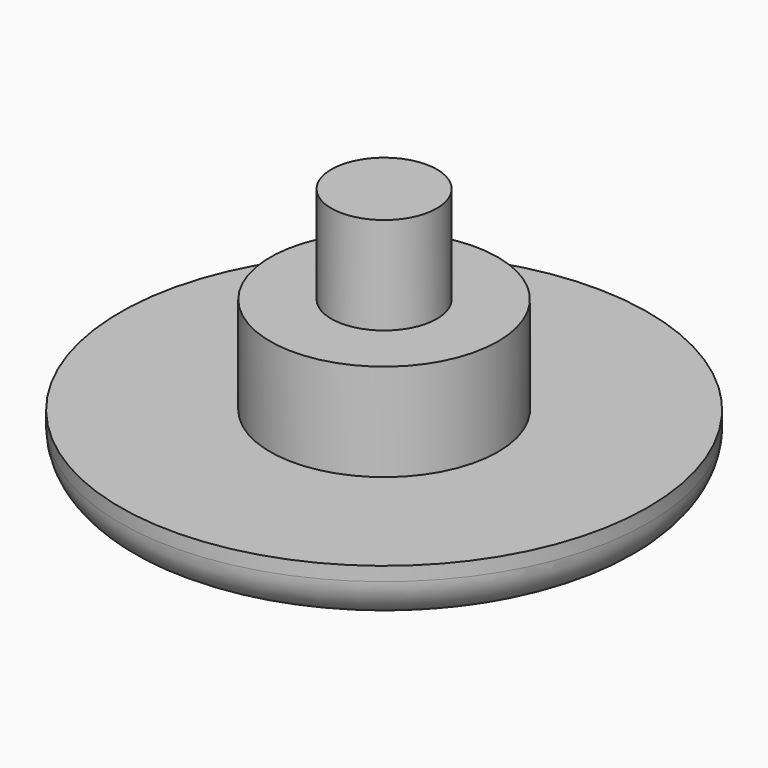
from build123d import *

# Parameters (mm, degrees)
F0_R     = 9.5
F0_R_2   = 4.1
F0_R_3   = 1.9
F1_DEPTH = 2
F2_R     = 4.1
F2_R_2   = 1.9
F3_DEPTH = 5.5
F4_R     = 1.5
F7_DEPTH = 7


# Not quite as in the source:
# - a feature names something its author has since deleted; it is built from what else it names


with BuildPart() as f1:
    # F0 (on Top) → F1 (new body)
    with BuildSketch(Plane.XY):
        Circle(F0_R)
        Circle(F0_R_2, mode=Mode.SUBTRACT)
        Circle(F0_R_2)
        Circle(F0_R_3, mode=Mode.SUBTRACT)
        Circle(F0_R_3)
    extrude(amount=F1_DEPTH)

    # F2 (on Top) → F3 (join)
    with BuildSketch(Plane.XY):
        Circle(F2_R)
        Circle(F2_R_2, mode=Mode.SUBTRACT)
    extrude(amount=F3_DEPTH)

    # F4
    f4_edges = [f1.edges().sort_by_distance(p)[0] for p in [
        (-9.5, 0, 0),
    ]]
    fillet(f4_edges, radius=F4_R)

    # F5 (on Front) → F6 (revolve, cut)
    with BuildSketch(Plane.XZ):
        with BuildLine():
            ThreePointArc((0, 0), (23.1570723538, -9.489364109), (32.9962119038, -32.5))
            ThreePointArc((32.9962119038, -32.5), (23.510635891, -8.8429276462), (0, 1))
            Line((0, 1), (0, 0))
        make_face()
    revolve(axis=Axis((0, 0, -31.5146126637), (0, 0, -1)), mode=Mode.SUBTRACT)

    # F7 (add): a face of the model
    f7_faces = [f1.faces().sort_by_distance(p)[0] for p in [
        (0, 0, 2),
    ]]
    extrude(f7_faces, amount=F7_DEPTH)


solid = f1.part
